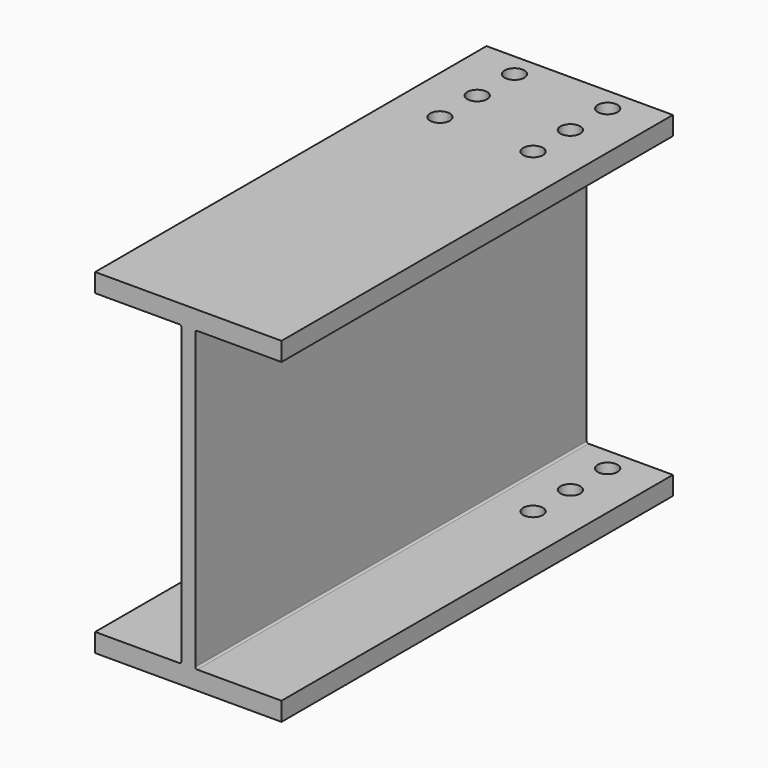
from build123d import *

# Parameters (mm, degrees)
F1_DEPTH      = 508
F1_DEPTH_BACK = 158.75
F3_D          = 26.9875
F3_DEPTH      = 25.4
F3_TIP        = 8.107862978
F5_D          = 26.9875
F5_DEPTH      = 25.4
F5_TIP        = 8.107862978


# Not quite as in the source:
# - a feature names something its author has since deleted; it is built from what else it names


with BuildPart() as f1:
    # F0 (on Front) → F1 (new body, two sides)
    with BuildSketch(Plane.XZ) as f1_sk:
        with BuildLine():
            Line((127, -228.6), (127, -203.2))
            Line((127, -203.2), (12.065, -203.2))
            ThreePointArc((12.065, -203.2), (10.2689487758, -202.4560512242), (9.525, -200.66))
            Line((9.525, -200.66), (9.525, 200.66))
            ThreePointArc((9.525, 200.66), (10.2689487758, 202.4560512242), (12.065, 203.2))
            Line((12.065, 203.2), (127, 203.2))
            Line((127, 203.2), (127, 228.6))
            Line((127, 228.6), (-127, 228.6))
            Line((-127, 228.6), (-127, 203.2))
            Line((-127, 203.2), (-12.065, 203.2))
            ThreePointArc((-12.065, 203.2), (-10.2689487758, 202.4560512242), (-9.525, 200.66))
            Line((-9.525, 200.66), (-9.525, -200.66))
            ThreePointArc((-9.525, -200.66), (-10.2689487758, -202.4560512242), (-12.065, -203.2))
            Line((-12.065, -203.2), (-127, -203.2))
            Line((-127, -203.2), (-127, -228.6))
            Line((-127, -228.6), (127, -228.6))
        make_face()
    extrude(amount=F1_DEPTH)
    extrude(f1_sk.sketch, amount=-F1_DEPTH_BACK)

    # F3
    with Locations(Plane.XY.offset(228.6)):
        with Locations((63.5, 127), (63.5, 63.5), (63.5, 0), (-63.5, 0), (-63.5, 63.5), (-63.5, 127)):
            Hole(F3_D / 2, depth=F3_DEPTH)
            with Locations((0, 0, -(F3_DEPTH + F3_TIP / 2))):  # 118° drill point
                Cone(0, F3_D / 2, F3_TIP, mode=Mode.SUBTRACT)

    # F5
    with Locations(Plane(origin=(0, 0, -228.6), x_dir=(1, 0, 0), z_dir=(0, 0, -1))):
        with Locations((63.5, -127), (63.5, -63.5), (63.5, 0), (-63.5, 0), (-63.5, -63.5), (-63.5, -127)):
            Hole(F5_D / 2, depth=F5_DEPTH)
            with Locations((0, 0, -(F5_DEPTH + F5_TIP / 2))):  # 118° drill point
                Cone(0, F5_D / 2, F5_TIP, mode=Mode.SUBTRACT)


solid = f1.part
